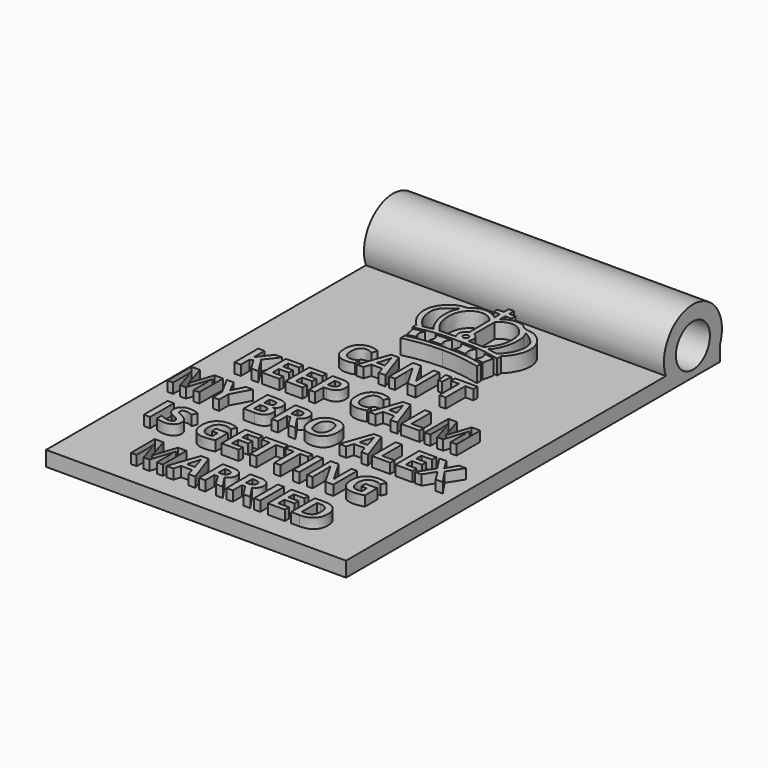
from build123d import *

# Parameters (mm, degrees)
F0_TEXT_SIZE = 8.3333333333
F2_DEPTH     = 2
F1_W         = 60
F1_H         = 80
F3_DEPTH     = 3
F5_DEPTH     = 3
F6_R         = 4.25
F7_DEPTH     = 60


# Not quite as in the source:
# - Text() gives the source's letters only with a copy of the font that has no kerning and outlines rounded to 1/6400 em; it was checked with that copy


with BuildPart() as f2:
    # F0 (on Top) → F2 (new body)
    with BuildSketch(Plane.XY):
        with Locations((18.5626573851, -3.6861407997)):
            Text("CAN'T", F0_TEXT_SIZE, font='Open Sans', font_style=FontStyle.BOLD, text_align=(TextAlign.LEFT, TextAlign.BOTTOM))
        with Locations((7.7358344684, -15.0194741331)):
            Text('KEEP CALM', F0_TEXT_SIZE, font='Open Sans', font_style=FontStyle.BOLD, text_align=(TextAlign.LEFT, TextAlign.BOTTOM))
        with Locations((3.4051053017, -26.3528074664)):
            Text('MY BRO ALEX', F0_TEXT_SIZE, font='Open Sans', font_style=FontStyle.BOLD, text_align=(TextAlign.LEFT, TextAlign.BOTTOM))
        with Locations((7.7358344684, -37.6861407997)):
            Text('IS GETTING', F0_TEXT_SIZE, font='Open Sans', font_style=FontStyle.BOLD, text_align=(TextAlign.LEFT, TextAlign.BOTTOM))
        with Locations((14.2319282184, -49.0194741331)):
            Text('MARRIED', F0_TEXT_SIZE, font='Open Sans', font_style=FontStyle.BOLD, text_align=(TextAlign.LEFT, TextAlign.BOTTOM))
    extrude(amount=F2_DEPTH)


with BuildPart() as f3:
    # F1 (on Top) → F3 (new body)
    with BuildSketch(Plane.XY):
        with Locations((31.6023485192, -13.5257663723)):
            Rectangle(F1_W, F1_H)
    extrude(amount=-F3_DEPTH)

    # F4 (on Top) → F5 (join)
    with BuildSketch(Plane.XY):
        with BuildLine():
            add(Edge.make_bspline(
                [(40.061801672, 6.1162402853), (39.4042474825, 6.2445407525), (38.0346070719, 6.5117818521), (35.6789580455, 6.9624974953), (33.5727332117, 7.0249018094), (32.4352048346, 7.0586050861)],
                knots=[0, 0, 0, 0, 0.2980976949, 0.6209171133, 1, 1, 1, 1], degree=3))
            Line((40.061801672, 6.1162402853), (40.061801672, 7.142174989))
            add(Edge.make_bspline(
                [(40.061801672, 7.142174989), (39.5391284737, 7.2667037), (38.3924908574, 7.539894108), (36.062554957, 7.8778935389), (33.7678631064, 7.9478965676), (32.8344636097, 7.958159267), (32.4352048346, 7.9625491053)],
                knots=[0, 0, 0, 0, 0.2357761128, 0.5172443524, 0.7935027508, 1, 1, 1, 1], degree=3))
            add(Edge.make_bspline(
                [(24.8086079972, 7.142174989), (25.3312811955, 7.2667037), (26.4779188118, 7.539894108), (28.8078547122, 7.8778935389), (31.1025465628, 7.9478965676), (32.0359460596, 7.958159267), (32.4352048346, 7.9625491053)],
                knots=[0, 0, 0, 0, 0.2357761128, 0.5172443524, 0.7935027508, 1, 1, 1, 1], degree=3))
            Line((24.8086079972, 7.142174989), (24.8086079972, 6.1162402853))
            add(Edge.make_bspline(
                [(24.8086079972, 6.1162402853), (25.4661621867, 6.2445407525), (26.8358025973, 6.5117818521), (29.1914516237, 6.9624974953), (31.2976764576, 7.0249018094), (32.4352048346, 7.0586050861)],
                knots=[0, 0, 0, 0, 0.2980976949, 0.6209171133, 1, 1, 1, 1], degree=3))
        make_face()
        with BuildLine():
            Line((36.566849798, 10.4196621105), (33.3498120308, 10.6030171737))
            add(Edge.make_bspline(
                [(33.7076857686, 8.3829201758), (33.7628695344, 8.5386566738), (33.8796338681, 8.8681823625), (34.0955873569, 9.5062059595), (33.7258304566, 10.1834878598), (33.4697817194, 10.4691652194), (33.3498120308, 10.6030171737)],
                knots=[0, 0, 0, 0, 0.22961142, 0.4858389796, 0.759093764, 1, 1, 1, 1], degree=3))
            Line((33.7076857686, 8.3829201758), (36.06678918, 8.2694143057))
            add(Edge.make_bspline(
                [(36.566849798, 10.4196621105), (36.381972045, 10.3004914582), (35.9967028702, 10.0521501724), (35.7592121446, 9.2426008075), (35.9594130535, 8.6091568251), (36.06678918, 8.2694143057)],
                knots=[0, 0, 0, 0, 0.2996037448, 0.6243481744, 1, 1, 1, 1], degree=3))
        make_face()
        with BuildLine():
            add(Edge.make_bspline(
                [(38.385535875, 10.1739839883), (38.5629202998, 9.9130943627), (38.9096907809, 9.4030787788), (38.750018356, 8.5031832983), (38.428232451, 8.1479464742), (38.2744558156, 7.9781841487)],
                knots=[0, 0, 0, 0, 0.353491141, 0.6910431578, 1, 1, 1, 1], degree=3))
            Line((38.2744558156, 7.9781841487), (40.0323346257, 7.604167331))
            Line((40.0323346257, 7.604167331), (40.484103382, 9.7274802042))
            Line((40.484103382, 9.7274802042), (38.385535875, 10.1739839883))
        make_face()
        with BuildLine():
            add(Edge.make_bspline(
                [(40.9088097513, 10.1070478559), (40.0690716633, 10.3013933421), (38.3134659034, 10.7077034283), (35.1576868132, 11.0679406459), (33.3196784679, 11.003676197), (32.4352048346, 10.9727513045)],
                knots=[0, 0, 0, 0, 0.3223388938, 0.6739006206, 1, 1, 1, 1], degree=3))
            Line((40.9088097513, 10.1070478559), (40.9088097513, 11.0916979611))
            add(Edge.make_bspline(
                [(40.9088097513, 11.0916979611), (41.1996807969, 11.3834264908), (41.9028327565, 12.0886513332), (43.268419716, 14.579776467), (43.0538123141, 17.911704657), (40.2966871632, 20.6545192375), (37.9317768969, 20.4557412765), (37.1520374327, 21.53554442), (35.571137023, 21.8267675429), (33.9640516601, 21.5371938351), (32.9226452006, 20.6345055312), (32.9612271379, 20.7951868963), (32.969329507, 20.8289306611)],
                knots=[0, 0, 0, 0, 0.0902703108, 0.2182195404, 0.3575521915, 0.5043500614, 0.6170349694, 0.7001994019, 0.794994713, 0.8990969434, 0.9788099323, 1, 1, 1, 1], degree=3))
            Line((32.969329507, 20.8289306611), (32.969329507, 22.0562182367))
            Line((32.969329507, 22.0562182367), (34.2195890853, 22.0562182367))
            Line((34.2195890853, 22.0562182367), (34.2195890853, 23.0645537376))
            Line((34.2195890853, 23.0645537376), (32.969329507, 23.0645537376))
            Line((32.969329507, 23.0645537376), (32.969329507, 24.2627486587))
            Line((32.969329507, 24.2627486587), (32.4352048346, 24.2627486587))
            Line((32.4352048346, 24.2627486587), (31.9010801622, 24.2627486587))
            Line((31.9010801622, 24.2627486587), (31.9010801622, 23.0645537376))
            Line((31.9010801622, 23.0645537376), (30.650820584, 23.0645537376))
            Line((30.650820584, 23.0645537376), (30.650820584, 22.0562182367))
            Line((30.650820584, 22.0562182367), (31.9010801622, 22.0562182367))
            Line((31.9010801622, 22.0562182367), (31.9010801622, 20.8289306611))
            add(Edge.make_bspline(
                [(23.961599918, 11.0916979611), (23.6707288723, 11.3834264908), (22.9675769127, 12.0886513332), (21.6019899532, 14.579776467), (21.8165973552, 17.911704657), (24.573722506, 20.6545192375), (26.9386327724, 20.4557412765), (27.7183722365, 21.53554442), (29.2992726463, 21.8267675429), (30.9063580091, 21.5371938351), (31.9477644687, 20.6345055312), (31.9091825314, 20.7951868963), (31.9010801622, 20.8289306611)],
                knots=[0, 0, 0, 0, 0.0902703108, 0.2182195404, 0.3575521915, 0.5043500614, 0.6170349694, 0.7001994019, 0.794994713, 0.8990969434, 0.9788099323, 1, 1, 1, 1], degree=3))
            Line((23.961599918, 11.0916979611), (23.961599918, 10.1070478559))
            add(Edge.make_bspline(
                [(23.961599918, 10.1070478559), (24.801338006, 10.3013933421), (26.5569437658, 10.7077034283), (29.712722856, 11.0679406459), (31.5507312013, 11.003676197), (32.4352048346, 10.9727513045)],
                knots=[0, 0, 0, 0, 0.3223388938, 0.6739006206, 1, 1, 1, 1], degree=3))
        make_face()
        with BuildLine():
            ThreePointArc((32.4352048346, 13.4262208926), (32.9824079867, 12.8790177405), (32.4352048346, 12.3318145884))
            ThreePointArc((32.4352048346, 12.3318145884), (31.8880016825, 12.8790177405), (32.4352048346, 13.4262208926))
        make_face(mode=Mode.SUBTRACT)
        with BuildLine():
            Line((26.9744023698, 11.6995451972), (25.0378623622, 11.352702044))
            add(Edge.make_bspline(
                [(25.0378623622, 11.352702044), (24.7211901731, 11.6494439082), (23.9921691064, 12.3325827433), (22.8191010768, 14.4227707179), (22.762786915, 16.7745279675), (23.6224159763, 18.234380741), (25.9647774401, 19.7913232511), (25.671775012, 19.2406416248), (25.1893662717, 18.2971727114), (25.1465321299, 16.8588695178), (25.15294801, 15.31293469), (26.1173678615, 12.6279128018), (26.7299207806, 11.9643755922), (26.9744023698, 11.6995451972)],
                knots=[0, 0, 0, 0, 0.0854782567, 0.1967821994, 0.3041400433, 0.4037933185, 0.5117480166, 0.5454076297, 0.6209341051, 0.7069101398, 0.7988588214, 0.9197207074, 1, 1, 1, 1], degree=3))
        make_face(mode=Mode.SUBTRACT)
        with BuildLine():
            Line((31.2413097751, 11.9259180822), (28.0464850383, 11.8157686666))
            add(Edge.make_bspline(
                [(31.9191329199, 19.4688625634), (31.6521422667, 19.755429734), (31.0696526846, 20.3806291162), (29.3336263214, 20.9054670146), (27.584519937, 20.2099904721), (26.3698311374, 18.7458985489), (25.9985060212, 16.9825511121), (26.0743894918, 14.7621084799), (26.9999536741, 13.0201170508), (27.7099389333, 12.2030659533), (28.0464850383, 11.8157686666)],
                knots=[0, 0, 0, 0, 0.1044214935, 0.2278148369, 0.3549685182, 0.4825287333, 0.6088104126, 0.7490369962, 0.8810389084, 1, 1, 1, 1], degree=3))
            Line((31.9191329199, 19.4688625634), (31.9577281223, 14.3301553497))
            ThreePointArc((31.9577281223, 14.3301553497), (30.9711487874, 13.3152794305), (31.2413097751, 11.9259180822))
        make_face(mode=Mode.SUBTRACT)
        with BuildLine():
            Line((32.9126815469, 14.3301553497), (32.9512767494, 19.4688625634))
            add(Edge.make_bspline(
                [(32.9512767494, 19.4688625634), (33.2182674026, 19.755429734), (33.8007569846, 20.3806291162), (35.5367833479, 20.9054670146), (37.2858897322, 20.2099904721), (38.5005785318, 18.7458985489), (38.871903648, 16.9825511121), (38.7960201774, 14.7621084799), (37.8704559951, 13.0201170508), (37.1604707359, 12.2030659533), (36.8239246309, 11.8157686666)],
                knots=[0, 0, 0, 0, 0.1044214935, 0.2278148369, 0.3549685182, 0.4825287333, 0.6088104126, 0.7490369962, 0.8810389084, 1, 1, 1, 1], degree=3))
            Line((36.8239246309, 11.8157686666), (33.6290998941, 11.9259180822))
            ThreePointArc((33.6290998941, 11.9259180822), (33.8992608819, 13.3152794305), (32.9126815469, 14.3301553497))
        make_face(mode=Mode.SUBTRACT)
        with BuildLine():
            Line((39.832547307, 11.352702044), (37.8960072994, 11.6995451972))
            add(Edge.make_bspline(
                [(39.832547307, 11.352702044), (40.1492194962, 11.6494439082), (40.8782405628, 12.3325827433), (42.0513085925, 14.4227707179), (42.1076227543, 16.7745279675), (41.2479936929, 18.234380741), (38.9056322291, 19.7913232511), (39.1986346573, 19.2406416248), (39.6810433976, 18.2971727114), (39.7238775394, 16.8588695178), (39.7174616592, 15.31293469), (38.7530418077, 12.6279128018), (38.1404888887, 11.9643755922), (37.8960072994, 11.6995451972)],
                knots=[0, 0, 0, 0, 0.0854782567, 0.1967821994, 0.3041400433, 0.4037933185, 0.5117480166, 0.5454076297, 0.6209341051, 0.7069101398, 0.7988588214, 0.9197207074, 1, 1, 1, 1], degree=3))
        make_face(mode=Mode.SUBTRACT)
        with BuildLine():
            Line((24.8380750435, 7.604167331), (26.5959538537, 7.9781841487))
            add(Edge.make_bspline(
                [(26.4848737942, 10.1739839883), (26.3074893694, 9.9130943627), (25.9607188883, 9.4030787788), (26.1203913132, 8.5031832983), (26.4421772183, 8.1479464742), (26.5959538537, 7.9781841487)],
                knots=[0, 0, 0, 0, 0.353491141, 0.6910431578, 1, 1, 1, 1], degree=3))
            Line((26.4848737942, 10.1739839883), (24.3863062872, 9.7274802042))
            Line((24.3863062872, 9.7274802042), (24.8380750435, 7.604167331))
        make_face()
        with BuildLine():
            add(Edge.make_bspline(
                [(28.3035598713, 10.4196621105), (28.4884376242, 10.3004914582), (28.873706799, 10.0521501724), (29.1111975246, 9.2426008075), (28.9109966157, 8.6091568251), (28.8036204892, 8.2694143057)],
                knots=[0, 0, 0, 0, 0.2996037448, 0.6243481744, 1, 1, 1, 1], degree=3))
            Line((28.8036204892, 8.2694143057), (31.1627239006, 8.3829201758))
            add(Edge.make_bspline(
                [(31.1627239006, 8.3829201758), (31.1075401348, 8.5386566738), (30.9907758011, 8.8681823625), (30.7748223124, 9.5062059595), (31.1445792126, 10.1834878598), (31.4006279498, 10.4691652194), (31.5205976384, 10.6030171737)],
                knots=[0, 0, 0, 0, 0.22961142, 0.4858389796, 0.759093764, 1, 1, 1, 1], degree=3))
            Line((31.5205976384, 10.6030171737), (28.3035598713, 10.4196621105))
        make_face()
    extrude(amount=F5_DEPTH)

    # F6 (on face) → F7 (join)
    with BuildSketch(Plane.YZ.offset(61.6023485192)):
        with BuildLine():
            Line((39.9676516476, -3), (39.9676516476, 0))
            ThreePointArc((39.9676516476, 0), (33.2077103853, 9.8702469599), (26.447769123, 0))
            Line((26.447769123, 0), (26.4742336277, 0))
            Line((26.4742336277, 0), (26.4742336277, -3))
            Line((26.4742336277, -3), (39.9676516476, -3))
        make_face()
        with Locations((33.2077103853, 2.6202469599)):
            Circle(F6_R, mode=Mode.SUBTRACT)
    extrude(amount=-F7_DEPTH)


solid = Compound([f2.part, f3.part])
